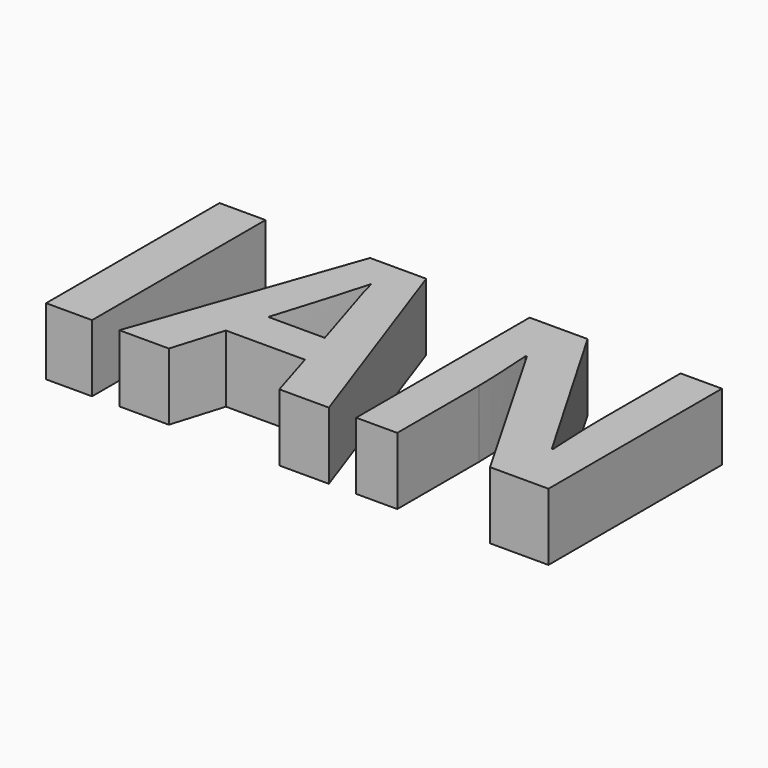
from build123d import *

# Parameters (mm, degrees)
F0_TEXT_SIZE = 114.9708560357
F1_DEPTH     = 25.4


# Not quite as in the source:
# - Text() gives the source's letters only with a copy of the font that has no kerning and outlines rounded to 1/6400 em; it was checked with that copy


with BuildPart() as f1:
    # F0 (on Top) → F1 (new body)
    with BuildSketch(Plane.XY):
        with Locations((-103.1822934747, -47.0732785761)):
            Text('IAN', F0_TEXT_SIZE, font='Open Sans', font_style=FontStyle.BOLD, text_align=(TextAlign.LEFT, TextAlign.BOTTOM))
    extrude(amount=F1_DEPTH)


solid = f1.part
